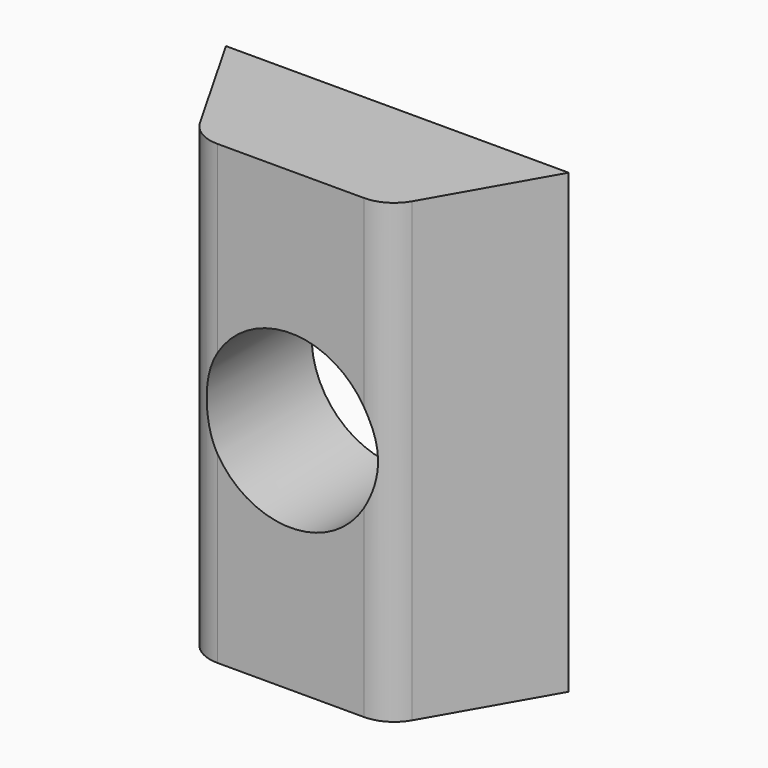
from build123d import *

# Parameters (mm, degrees)
F1_DEPTH    = 12
F3_D        = 4.5
F4_T1_DEPTH = 14.9016126774


# Not quite as in the source:
# - a fillet or chamfer that OpenCascade refuses, or shapes differently, is made with other operations: its cross-section is extruded or revolved along the edge and cut away or added


with BuildPart() as f1:
    # F0 (on Top) → F1 (new body)
    with BuildSketch(Plane.XY):
        Polygon((-2.5, -1.75), (2.5, -1.75), (4.5, 1.75), (-4.5, 1.75), align=None)
    extrude(amount=F1_DEPTH)

    # F3 (through all)
    with Locations(Plane(origin=(0, 1.75, 0), x_dir=(-1, 0, 0), z_dir=(0, 1, 0))):
        with Locations((0, 6)):
            Hole(F3_D / 2)

    # F4: fillet of radius 1 on 2 edges, made by hand

    # F4_s2 → F4_t1 (cut)
    with BuildSketch(Plane.XY.offset(-1.4508063387)):
        with BuildLine():
            ThreePointArc((1.9196774645, -1.75), (2.4216042827, -1.6149100931), (2.7879206067, -1.2461389384))
            Line((2.7879206067, -1.2461389384), (2.5, -1.75))
            Line((2.5, -1.75), (1.9196774645, -1.75))
        make_face()
        with BuildLine():
            ThreePointArc((-1.9196774645, -1.75), (-2.4216042827, -1.6149100931), (-2.7879206067, -1.2461389384))
            Line((-2.7879206067, -1.2461389384), (-2.5, -1.75))
            Line((-2.5, -1.75), (-1.9196774645, -1.75))
        make_face()
    extrude(amount=F4_T1_DEPTH, mode=Mode.SUBTRACT)


solid = f1.part
